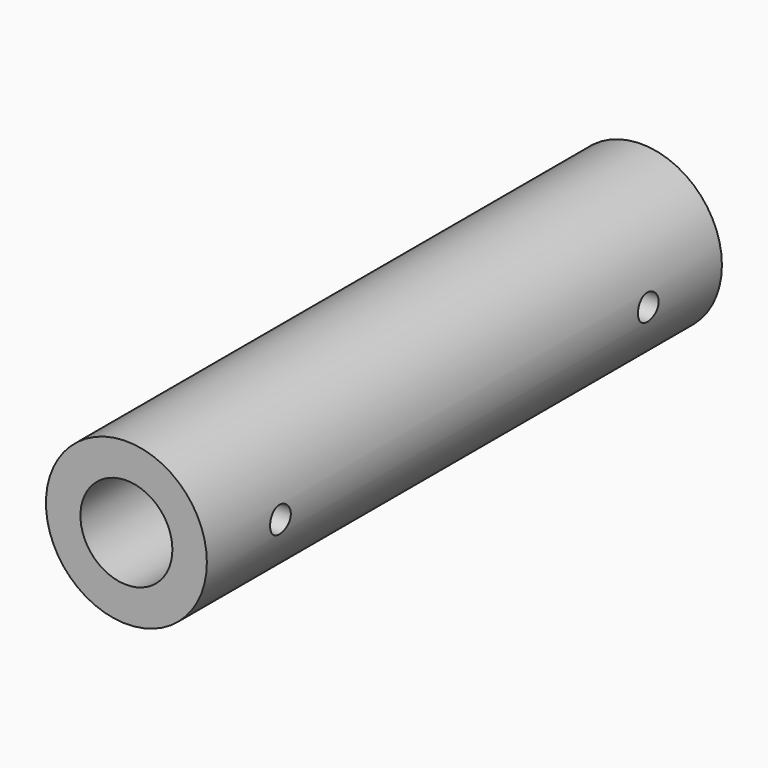
from build123d import *

# Parameters (mm, degrees)
F0_R     = 11.1125
F0_R_2   = 6.35
F1_DEPTH = 44.45
F2_R     = 1.7907
F3_DEPTH = 12.7


# Not quite as in the source:
# - a pattern or mirror of a feature is missing from the dataset's text; its kind, count and spacing are read off the source's solid


with BuildPart() as f1:
    # F0 (on Front) → F1 (new body, symmetric)
    with BuildSketch(Plane.XZ):
        Circle(F0_R)
        Circle(F0_R_2, mode=Mode.SUBTRACT)
    extrude(amount=F1_DEPTH, both=True)

    # F2 (on Right) → F3 (cut)
    with BuildSketch(Plane.YZ):
        with Locations((-31.75, 0)):
            Circle(F2_R)
    f3 = extrude(amount=F3_DEPTH, mode=Mode.SUBTRACT)

    # F3_copies: F3 across plane
    add(f3.mirror(Plane.ZX), mode=Mode.SUBTRACT)


solid = f1.part
